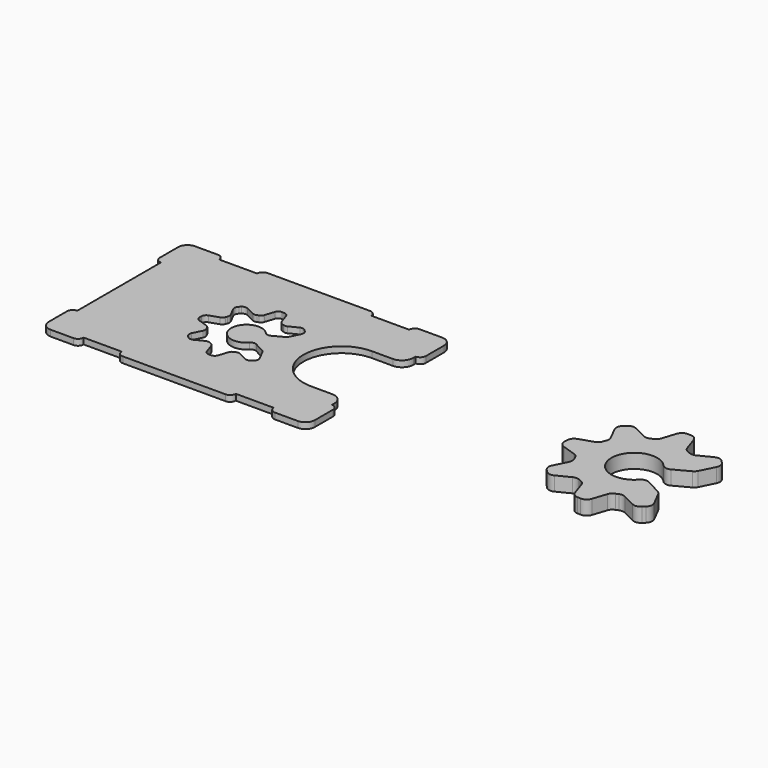
from build123d import *

# Parameters (mm, degrees)
F1_DEPTH = 2.032
F4_DEPTH = 25.4
F5_DEPTH = 3.175
F6_SCALE = 1.5
F7_R     = 1.90499
F8_R     = 3.81


# Not quite as in the source:
# - a fillet or chamfer is up to 0.001 mm smaller than in the source, because OpenCascade refuses the exact size


with BuildPart() as f1:
    # F0 (on Top) → F1 (new body)
    with BuildSketch(Plane.XY):
        with BuildLine():
            Line((31.75, -30.1625), (41.275, -30.1625))
            ThreePointArc((41.275, -30.1625), (43.5200640303, -29.2325640303), (44.45, -26.9875))
            Line((44.45, -26.9875), (44.45, -17.4625))
            Line((44.45, -17.4625), (42.545, -17.4625))
            Line((42.545, -17.4625), (42.545, -12.7))
            Line((42.545, -12.7), (31.75, -12.7))
            ThreePointArc((31.75, -12.7), (19.05, 0), (31.75, 12.7))
            Line((31.75, 12.7), (42.545, 12.7))
            Line((42.545, 12.7), (42.545, 17.4625))
            Line((42.545, 17.4625), (44.45, 17.4625))
            Line((44.45, 17.4625), (44.45, 26.9875))
            ThreePointArc((44.45, 26.9875), (43.5200640303, 29.2325640303), (41.275, 30.1625))
            Line((41.275, 30.1625), (31.75, 30.1625))
            Line((31.75, 30.1625), (31.75, 28.2575))
            Line((31.75, 28.2575), (19.05, 28.2575))
            Line((19.05, 28.2575), (19.05, 30.1625))
            Line((19.05, 30.1625), (-19.05, 30.1625))
            Line((-19.05, 30.1625), (-19.05, 28.2575))
            Line((-19.05, 28.2575), (-31.75, 28.2575))
            Line((-31.75, 28.2575), (-31.75, 30.1625))
            Line((-31.75, 30.1625), (-41.275, 30.1625))
            ThreePointArc((-41.275, 30.1625), (-43.5200640303, 29.2325640303), (-44.45, 26.9875))
            Line((-44.45, 26.9875), (-44.45, 17.4625))
            Line((-44.45, 17.4625), (-42.545, 17.4625))
            Line((-42.545, 17.4625), (-42.545, -17.4625))
            Line((-42.545, -17.4625), (-44.45, -17.4625))
            Line((-44.45, -17.4625), (-44.45, -26.9875))
            ThreePointArc((-44.45, -26.9875), (-43.5200640303, -29.2325640303), (-41.275, -30.1625))
            Line((-41.275, -30.1625), (-31.75, -30.1625))
            Line((-31.75, -30.1625), (-31.75, -28.2575))
            Line((-31.75, -28.2575), (-19.05, -28.2575))
            Line((-19.05, -28.2575), (-19.05, -30.1625))
            Line((-19.05, -30.1625), (19.05, -30.1625))
            Line((19.05, -30.1625), (19.05, -28.2575))
            Line((19.05, -28.2575), (31.75, -28.2575))
            Line((31.75, -28.2575), (31.75, -30.1625))
        make_face()
    extrude(amount=F1_DEPTH)

    # F2 (on face) → F4 (cut)
    with BuildSketch(Plane.XY.offset(2.032)):
        with BuildLine():
            Line((9.7686970333, 5.5580902606), (11.3443342276, 8.7233058886))
            ThreePointArc((11.3443342276, 8.7233058886), (11.4949714702, 9.6693211472), (11.078264348, 10.5318706372))
            Line((11.078264348, 10.5318706372), (10.5976845378, 11.0435955275))
            ThreePointArc((10.5976845378, 11.0435955275), (9.7075030286, 11.5243078851), (8.7068940027, 11.375012649))
            Line((8.7068940027, 11.375012649), (5.8087867996, 9.903819134))
            ThreePointArc((5.8087867996, 9.903819134), (5.1228026077, 9.7309544558), (4.4293224067, 9.8707461557))
            ThreePointArc((4.4293224067, 9.8707461557), (4.1354631897, 9.997423211), (3.8379861099, 10.1153541348))
            ThreePointArc((3.8379861099, 10.1153541348), (3.2522185144, 10.5023214943), (2.8884612744, 11.1027780568))
            Line((2.8884612744, 11.1027780568), (1.8533469122, 14.1899644085))
            ThreePointArc((1.8533469122, 14.1899644085), (1.2909297235, 14.9654148287), (0.3863586981, 15.2806729904))
            Line((0.3863586981, 15.2806729904), (-0.3153066846, 15.3026958878))
            ThreePointArc((-0.3153066846, 15.3026958878), (-1.2846750341, 15.0131574739), (-1.8866447878, 14.2000523726))
            Line((-1.8866447878, 14.2000523726), (-2.8956251329, 11.1104902057))
            ThreePointArc((-2.8956251329, 11.1104902057), (-3.2584554205, 10.5031923457), (-3.8476676322, 10.1116754519))
            ThreePointArc((-3.8476676322, 10.1116754519), (-4.1450316821, 9.9934598117), (-4.4387694984, 9.8665015073))
            ThreePointArc((-4.4387694984, 9.8665015073), (-5.1265969814, 9.7259285122), (-5.8083990997, 9.8933002083))
            Line((-5.8083990997, 9.8933002083), (-8.7233058886, 11.3443342276))
            ThreePointArc((-8.7233058886, 11.3443342276), (-9.6693211472, 11.4949714702), (-10.5318706372, 11.078264348))
            Line((-10.5318706372, 11.078264348), (-11.0435955275, 10.5976845378))
            ThreePointArc((-11.0435955275, 10.5976845378), (-11.5243078851, 9.7075030286), (-11.375012649, 8.7068940027))
            Line((-11.375012649, 8.7068940027), (-9.903819134, 5.8087867996))
            ThreePointArc((-9.903819134, 5.8087867996), (-9.7309544558, 5.1228026077), (-9.8707461557, 4.4293224067))
            ThreePointArc((-9.8707461557, 4.4293224067), (-9.997423211, 4.1354631897), (-10.1153541348, 3.8379861099))
            ThreePointArc((-10.1153541348, 3.8379861099), (-10.5023214943, 3.2522185144), (-11.1027780568, 2.8884612744))
            Line((-11.1027780568, 2.8884612744), (-14.1899644085, 1.8533469122))
            ThreePointArc((-14.1899644085, 1.8533469122), (-14.9654148287, 1.2909297235), (-15.2806729904, 0.3863586981))
            Line((-15.2806729904, 0.3863586981), (-15.3026958878, -0.3153066846))
            ThreePointArc((-15.3026958878, -0.3153066846), (-15.0131574739, -1.2846750341), (-14.2000523726, -1.8866447878))
            Line((-14.2000523726, -1.8866447878), (-11.1104902057, -2.8956251329))
            ThreePointArc((-11.1104902057, -2.8956251329), (-10.5031923457, -3.2584554205), (-10.1116754519, -3.8476676322))
            ThreePointArc((-10.1116754519, -3.8476676322), (-9.9934598117, -4.1450316821), (-9.8665015073, -4.4387694984))
            ThreePointArc((-9.8665015073, -4.4387694984), (-9.7259285122, -5.1265969814), (-9.8933002083, -5.8083990997))
            Line((-9.8933002083, -5.8083990997), (-11.3443342276, -8.7233058886))
            ThreePointArc((-11.3443342276, -8.7233058886), (-11.4949714702, -9.6693211472), (-11.078264348, -10.5318706372))
            Line((-11.078264348, -10.5318706372), (-10.5976845378, -11.0435955275))
            ThreePointArc((-10.5976845378, -11.0435955275), (-9.7075030286, -11.5243078851), (-8.7068940027, -11.375012649))
            Line((-8.7068940027, -11.375012649), (-5.8087867996, -9.903819134))
            ThreePointArc((-5.8087867996, -9.903819134), (-5.1228026077, -9.7309544558), (-4.4293224067, -9.8707461557))
            ThreePointArc((-4.4293224067, -9.8707461557), (-4.1354631897, -9.997423211), (-3.8379861099, -10.1153541348))
            ThreePointArc((-3.8379861099, -10.1153541348), (-3.2522185144, -10.5023214943), (-2.8884612744, -11.1027780568))
            Line((-2.8884612744, -11.1027780568), (-1.8533469122, -14.1899644085))
            ThreePointArc((-1.8533469122, -14.1899644085), (-1.2909297235, -14.9654148287), (-0.3863586981, -15.2806729904))
            Line((-0.3863586981, -15.2806729904), (0.3153066846, -15.3026958878))
            ThreePointArc((0.3153066846, -15.3026958878), (1.2846750341, -15.0131574739), (1.8866447878, -14.2000523726))
            Line((1.8866447878, -14.2000523726), (2.8956251329, -11.1104902057))
            ThreePointArc((2.8956251329, -11.1104902057), (3.2584554205, -10.5031923457), (3.8476676322, -10.1116754519))
            ThreePointArc((3.8476676322, -10.1116754519), (4.1450316821, -9.9934598117), (4.4387694984, -9.8665015073))
            ThreePointArc((4.4387694984, -9.8665015073), (5.1265969814, -9.7259285122), (5.8083990997, -9.8933002083))
            Line((5.8083990997, -9.8933002083), (8.7233058886, -11.3443342276))
            ThreePointArc((8.7233058886, -11.3443342276), (9.6693211472, -11.4949714702), (10.5318706372, -11.078264348))
            Line((10.5318706372, -11.078264348), (11.0435955275, -10.5976845378))
            ThreePointArc((11.0435955275, -10.5976845378), (11.5243078851, -9.7075030286), (11.375012649, -8.7068940027))
            Line((11.375012649, -8.7068940027), (9.7710078453, -5.5471615622))
            ThreePointArc((9.7710078453, -5.5471615622), (9.4873948591, -5.1518612931), (9.0981017728, -4.8600573835))
            Line((9.0981017728, -4.8600573835), (5.7308372239, -3.0613196532))
            ThreePointArc((5.7308372239, -3.0613196532), (4.6997765488, -2.8967353459), (3.7866854345, -3.4031331412))
            ThreePointArc((3.7866854345, -3.4031331412), (-5.0911983871, -0.0008598127), (3.7855357613, 3.4044119545))
            ThreePointArc((3.7855357613, 3.4044119545), (4.6987978667, 2.8983225977), (5.7298028923, 3.0632551512))
            Line((5.7298028923, 3.0632551512), (9.0906211871, 4.8600087477))
            ThreePointArc((9.0906211871, 4.8600087477), (9.4840151212, 5.1562512313), (9.7686970333, 5.5580902606))
        make_face()
    extrude(amount=-F4_DEPTH, mode=Mode.SUBTRACT)

    # F7 (radius 1.905 in the source; OpenCascade refuses exactly that, so slightly less here)
    f7_edges = [f1.edges().sort_by_distance(p)[0] for p in [
        (44.45, -17.4625, 1.016),
        (44.45, 17.4625, 1.016),
        (19.05, -30.1625, 1.016),
        (31.75, -30.1625, 1.016),
        (-31.75, -30.1625, 1.016),
        (-19.05, -30.1625, 1.016),
        (-44.45, -17.4625, 1.016),
        (-44.45, 17.4625, 1.016),
        (-19.05, 30.1625, 1.016),
        (-31.75, 30.1625, 1.016),
        (31.75, 30.1625, 1.016),
        (19.05, 30.1625, 1.016),
    ]]
    fillet(f7_edges, radius=F7_R)

    # F8
    f8_edges = [f1.edges().sort_by_distance(p)[0] for p in [
        (42.545, 12.7, 1.016),
        (42.545, -12.7, 1.016),
    ]]
    fillet(f8_edges, radius=F8_R)


with BuildPart() as f5:
    # F3 (on Top) → F5 (new body)
    with BuildSketch(Plane.XY):
        with BuildLine():
            Line((138.8378861171, 6.1610323828), (140.4135233114, 9.3262480107))
            ThreePointArc((140.4135233114, 9.3262480107), (140.5641605541, 10.2722632693), (140.1474534319, 11.1348127593))
            Line((140.1474534319, 11.1348127593), (139.6668736217, 11.6465376496))
            ThreePointArc((139.6668736217, 11.6465376496), (138.7766921125, 12.1272500072), (137.7760830866, 11.9779547711))
            Line((137.7760830866, 11.9779547711), (134.8779758834, 10.5067612561))
            ThreePointArc((134.8779758834, 10.5067612561), (134.1919916916, 10.3338965779), (133.4985114906, 10.4736882778))
            ThreePointArc((133.4985114906, 10.4736882778), (133.2046522736, 10.6003653331), (132.9071751938, 10.718296257))
            ThreePointArc((132.9071751938, 10.718296257), (132.3214075983, 11.1052636164), (131.9576503582, 11.705720179))
            Line((131.9576503582, 11.705720179), (130.9225359961, 14.7929065306))
            ThreePointArc((130.9225359961, 14.7929065306), (130.3601188074, 15.5683569509), (129.455547782, 15.8836151125))
            Line((129.455547782, 15.8836151125), (128.7538823993, 15.9056380099))
            ThreePointArc((128.7538823993, 15.9056380099), (127.7845140498, 15.616099596), (127.1825442961, 14.8029944947))
            Line((127.1825442961, 14.8029944947), (126.173563951, 11.7134323279))
            ThreePointArc((126.173563951, 11.7134323279), (125.8107336634, 11.1061344678), (125.2215214517, 10.7146175741))
            ThreePointArc((125.2215214517, 10.7146175741), (124.9241574018, 10.5964019338), (124.6304195854, 10.4694436294))
            ThreePointArc((124.6304195854, 10.4694436294), (123.9425921025, 10.3288706343), (123.2607899842, 10.4962423304))
            Line((123.2607899842, 10.4962423304), (120.3458831953, 11.9472763497))
            ThreePointArc((120.3458831953, 11.9472763497), (119.3998679367, 12.0979135923), (118.5373184467, 11.6812064701))
            Line((118.5373184467, 11.6812064701), (118.0255935564, 11.20062666))
            ThreePointArc((118.0255935564, 11.20062666), (117.5448811988, 10.3104451507), (117.6941764349, 9.3098361249))
            Line((117.6941764349, 9.3098361249), (119.1653699499, 6.4117289217))
            ThreePointArc((119.1653699499, 6.4117289217), (119.3382346281, 5.7257447298), (119.1984429282, 5.0322645289))
            ThreePointArc((119.1984429282, 5.0322645289), (119.0717658729, 4.7384053118), (118.953834949, 4.440928232))
            ThreePointArc((118.953834949, 4.440928232), (118.5668675896, 3.8551606365), (117.966411027, 3.4914033965))
            Line((117.966411027, 3.4914033965), (114.8792246754, 2.4562890343))
            ThreePointArc((114.8792246754, 2.4562890343), (114.1037742551, 1.8938718456), (113.7885160935, 0.9893008203))
            Line((113.7885160935, 0.9893008203), (113.7664931961, 0.2876354375))
            ThreePointArc((113.7664931961, 0.2876354375), (114.05603161, -0.681732912), (114.8691367113, -1.2837026656))
            Line((114.8691367113, -1.2837026656), (117.9586988782, -2.2926830107))
            ThreePointArc((117.9586988782, -2.2926830107), (118.5659967382, -2.6555132984), (118.957513632, -3.2447255101))
            ThreePointArc((118.957513632, -3.2447255101), (119.0757292722, -3.54208956), (119.2026875766, -3.8358273763))
            ThreePointArc((119.2026875766, -3.8358273763), (119.3432605717, -4.5236548592), (119.1758888756, -5.2054569776))
            Line((119.1758888756, -5.2054569776), (117.7248548563, -8.1203637664))
            ThreePointArc((117.7248548563, -8.1203637664), (117.5742176137, -9.066379025), (117.9909247359, -9.9289285151))
            Line((117.9909247359, -9.9289285151), (118.4715045461, -10.4406534054))
            ThreePointArc((118.4715045461, -10.4406534054), (119.3616860553, -10.9213657629), (120.3622950811, -10.7720705268))
            Line((120.3622950811, -10.7720705268), (123.2604022843, -9.3008770119))
            ThreePointArc((123.2604022843, -9.3008770119), (123.9463864762, -9.1280123336), (124.6398666772, -9.2678040336))
            ThreePointArc((124.6398666772, -9.2678040336), (124.9337258942, -9.3944810889), (125.231202974, -9.5124120127))
            ThreePointArc((125.231202974, -9.5124120127), (125.8169705695, -9.8993793721), (126.1807278095, -10.4998359347))
            Line((126.1807278095, -10.4998359347), (127.2158421717, -13.5870222864))
            ThreePointArc((127.2158421717, -13.5870222864), (127.7782593604, -14.3624727066), (128.6828303858, -14.6777308682))
            Line((128.6828303858, -14.6777308682), (129.3844957685, -14.6997537656))
            ThreePointArc((129.3844957685, -14.6997537656), (130.353864118, -14.4102153518), (130.9558338716, -13.5971102504))
            Line((130.9558338716, -13.5971102504), (131.9648142167, -10.5075480836))
            ThreePointArc((131.9648142167, -10.5075480836), (132.3276445044, -9.9002502235), (132.9168567161, -9.5087333298))
            ThreePointArc((132.9168567161, -9.5087333298), (133.214220766, -9.3905176895), (133.5079585823, -9.2635593851))
            ThreePointArc((133.5079585823, -9.2635593851), (134.1957860653, -9.1229863901), (134.8775881836, -9.2903580862))
            Line((134.8775881836, -9.2903580862), (137.7924949724, -10.7413921054))
            ThreePointArc((137.7924949724, -10.7413921054), (138.738510231, -10.892029348), (139.6010597211, -10.4753222259))
            Line((139.6010597211, -10.4753222259), (140.1127846114, -9.9947424157))
            ThreePointArc((140.1127846114, -9.9947424157), (140.593496969, -9.1045609064), (140.4442017329, -8.1039518806))
            Line((140.4442017329, -8.1039518806), (138.8401969291, -4.9442194401))
            ThreePointArc((138.8401969291, -4.9442194401), (138.556583943, -4.5489191709), (138.1672908567, -4.2571152614))
            Line((138.1672908567, -4.2571152614), (134.8000263078, -2.4583775311))
            ThreePointArc((134.8000263078, -2.4583775311), (133.7689656327, -2.2937932238), (132.8558745183, -2.800191019))
            ThreePointArc((132.8558745183, -2.800191019), (123.9779906968, 0.6020823094), (132.8547248452, 4.0073540766))
            ThreePointArc((132.8547248452, 4.0073540766), (133.7679869506, 3.5012647199), (134.7989919762, 3.6661972734))
            Line((134.7989919762, 3.6661972734), (138.159810271, 5.4629508698))
            ThreePointArc((138.159810271, 5.4629508698), (138.5532042051, 5.7591933534), (138.8378861171, 6.1610323828))
        make_face()
    extrude(amount=F5_DEPTH)


with BuildPart() as f5_1:
    # F6: moved
    add(f5.part.scale(F6_SCALE).moved(Location((-64.5345945418, -0.3014710609, 0))))


solid = Compound([f1.part, f5_1.part])
